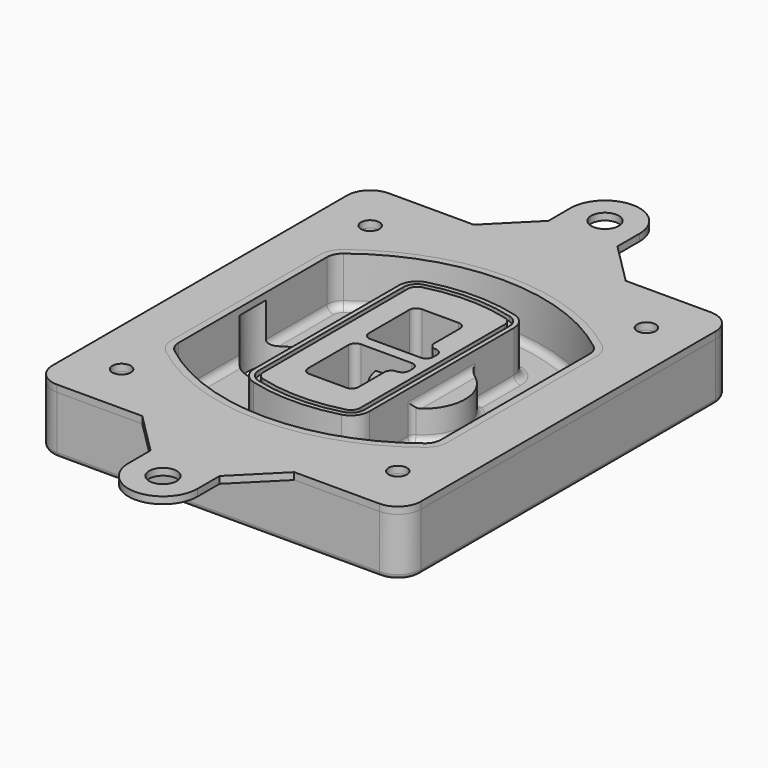
from build123d import *

# Parameters (mm, degrees)
F0_R      = 4
F1_DEPTH  = 25
F2_DEPTH  = 3
F3_DEPTH  = 18
F5_DEPTH  = 21
F6_DEPTH  = 2
F8_DEPTH  = 20
F9_DEPTH  = 16
F10_DEPTH = 25
F7_R      = 6
F7_R_2    = 4
F11_DEPTH = 6
F13_DEPTH = 9
F14_R     = 3
F15_R     = 2
F16_R     = 6
F16_R_2   = 4
F17_DEPTH = 3


# Not quite as in the source:
# - a feature names something its author has since deleted; it is built from what else it names


with BuildPart() as f1:
    # F0 (on Top) → F1 (new body)
    with BuildSketch(Plane.XY):
        with BuildLine():
            ThreePointArc((-80, -80), (-77.0710678119, -87.0710678119), (-70, -90))
            Line((-70, -90), (70, -90))
            ThreePointArc((70, -90), (77.0710678119, -87.0710678119), (80, -80))
            Line((80, -80), (80, 80))
            ThreePointArc((80, 80), (77.0710678119, 87.0710678119), (70, 90))
            Line((70, 90), (-70, 90))
            ThreePointArc((-70, 90), (-77.0710678119, 87.0710678119), (-80, 80))
            Line((-80, 80), (-80, -80))
        make_face()
        with Locations((-60, -67.5)):
            Circle(F0_R, mode=Mode.SUBTRACT)
        with Locations((60, -67.5)):
            Circle(F0_R, mode=Mode.SUBTRACT)
        with Locations((-60, 67.5)):
            Circle(F0_R, mode=Mode.SUBTRACT)
        with BuildLine():
            ThreePointArc((-64, 40.2934422872), (-62.5820384798, 46.4328484224), (-58.6153846154, 51.3286200352))
            ThreePointArc((-58.6153846154, 51.3286200352), (0, 71.5), (58.6153846154, 51.3286200352))
            ThreePointArc((58.6153846154, 51.3286200352), (62.5820384798, 46.4328484224), (64, 40.2934422872))
            Line((64, 40.2934422872), (64, -40.2934422872))
            ThreePointArc((64, -40.2934422872), (62.5820384798, -46.4328484224), (58.6153846154, -51.3286200352))
            ThreePointArc((58.6153846154, -51.3286200352), (0, -71.5), (-58.6153846154, -51.3286200352))
            ThreePointArc((-58.6153846154, -51.3286200352), (-62.5820384798, -46.4328484224), (-64, -40.2934422872))
            Line((-64, -40.2934422872), (-64, 40.2934422872))
        make_face(mode=Mode.SUBTRACT)
        with Locations((60, 67.5)):
            Circle(F0_R, mode=Mode.SUBTRACT)
        with BuildLine():
            ThreePointArc((58.6153846154, 51.3286200352), (0, 71.5), (-58.6153846154, 51.3286200352))
            ThreePointArc((-58.6153846154, 51.3286200352), (-62.5820384798, 46.4328484224), (-64, 40.2934422872))
            Line((-64, 40.2934422872), (-64, -40.2934422872))
            ThreePointArc((-64, -40.2934422872), (-62.5820384798, -46.4328484224), (-58.6153846154, -51.3286200352))
            ThreePointArc((-58.6153846154, -51.3286200352), (0, -71.5), (58.6153846154, -51.3286200352))
            ThreePointArc((58.6153846154, -51.3286200352), (62.5820384798, -46.4328484224), (64, -40.2934422872))
            Line((64, -40.2934422872), (64, 40.2934422872))
            ThreePointArc((64, 40.2934422872), (62.5820384798, 46.4328484224), (58.6153846154, 51.3286200352))
        make_face()
        with BuildLine():
            Line((-60, -40.2934422872), (-60, 40.2934422872))
            ThreePointArc((-60, 40.2934422872), (-58.9871703427, 44.6787323838), (-56.1538461538, 48.1757121072))
            ThreePointArc((-56.1538461538, 48.1757121072), (0, 67.5), (56.1538461538, 48.1757121072))
            ThreePointArc((56.1538461538, 48.1757121072), (58.9871703427, 44.6787323838), (60, 40.2934422872))
            Line((60, 40.2934422872), (60, -40.2934422872))
            ThreePointArc((60, -40.2934422872), (58.9871703427, -44.6787323838), (56.1538461538, -48.1757121072))
            ThreePointArc((56.1538461538, -48.1757121072), (0, -67.5), (-56.1538461538, -48.1757121072))
            ThreePointArc((-56.1538461538, -48.1757121072), (-58.9871703427, -44.6787323838), (-60, -40.2934422872))
        make_face(mode=Mode.SUBTRACT)
        with BuildLine():
            ThreePointArc((-56.1538461538, 48.1757121072), (-58.9871703427, 44.6787323838), (-60, 40.2934422872))
            Line((-60, 40.2934422872), (-60, -40.2934422872))
            ThreePointArc((-60, -40.2934422872), (-58.9871703427, -44.6787323838), (-56.1538461538, -48.1757121072))
            ThreePointArc((-56.1538461538, -48.1757121072), (0, -67.5), (56.1538461538, -48.1757121072))
            ThreePointArc((56.1538461538, -48.1757121072), (58.9871703427, -44.6787323838), (60, -40.2934422872))
            Line((60, -40.2934422872), (60, 40.2934422872))
            ThreePointArc((60, 40.2934422872), (58.9871703427, 44.6787323838), (56.1538461538, 48.1757121072))
            ThreePointArc((56.1538461538, 48.1757121072), (0, 67.5), (-56.1538461538, 48.1757121072))
        make_face()
        with BuildLine():
            ThreePointArc((54.3076923077, 45.8110311612), (56.2910192399, 43.3631453548), (57, 40.2934422872))
            Line((57, 40.2934422872), (57, -40.2934422872))
            ThreePointArc((57, -40.2934422872), (56.2910192399, -43.3631453548), (54.3076923077, -45.8110311612))
            ThreePointArc((54.3076923077, -45.8110311612), (0, -64.5), (-54.3076923077, -45.8110311612))
            ThreePointArc((-54.3076923077, -45.8110311612), (-56.2910192399, -43.3631453548), (-57, -40.2934422872))
            Line((-57, -40.2934422872), (-57, 40.2934422872))
            ThreePointArc((-57, 40.2934422872), (-56.2910192399, 43.3631453548), (-54.3076923077, 45.8110311612))
            ThreePointArc((-54.3076923077, 45.8110311612), (0, 64.5), (54.3076923077, 45.8110311612))
        make_face(mode=Mode.SUBTRACT)
        with BuildLine():
            Line((57, -40.2934422872), (57, 40.2934422872))
            ThreePointArc((57, 40.2934422872), (56.2910192399, 43.3631453548), (54.3076923077, 45.8110311612))
            ThreePointArc((54.3076923077, 45.8110311612), (0, 64.5), (-54.3076923077, 45.8110311612))
            ThreePointArc((-54.3076923077, 45.8110311612), (-56.2910192399, 43.3631453548), (-57, 40.2934422872))
            Line((-57, 40.2934422872), (-57, -40.2934422872))
            ThreePointArc((-57, -40.2934422872), (-56.2910192399, -43.3631453548), (-54.3076923077, -45.8110311612))
            ThreePointArc((-54.3076923077, -45.8110311612), (0, -64.5), (54.3076923077, -45.8110311612))
            ThreePointArc((54.3076923077, -45.8110311612), (56.2910192399, -43.3631453548), (57, -40.2934422872))
        make_face()
    extrude(amount=-F1_DEPTH)

    # F0 (on Top) → F2 (join)
    with BuildSketch(Plane.XY):
        with BuildLine():
            ThreePointArc((-56.1538461538, 48.1757121072), (-58.9871703427, 44.6787323838), (-60, 40.2934422872))
            Line((-60, 40.2934422872), (-60, -40.2934422872))
            ThreePointArc((-60, -40.2934422872), (-58.9871703427, -44.6787323838), (-56.1538461538, -48.1757121072))
            ThreePointArc((-56.1538461538, -48.1757121072), (0, -67.5), (56.1538461538, -48.1757121072))
            ThreePointArc((56.1538461538, -48.1757121072), (58.9871703427, -44.6787323838), (60, -40.2934422872))
            Line((60, -40.2934422872), (60, 40.2934422872))
            ThreePointArc((60, 40.2934422872), (58.9871703427, 44.6787323838), (56.1538461538, 48.1757121072))
            ThreePointArc((56.1538461538, 48.1757121072), (0, 67.5), (-56.1538461538, 48.1757121072))
        make_face()
        with BuildLine():
            ThreePointArc((54.3076923077, 45.8110311612), (56.2910192399, 43.3631453548), (57, 40.2934422872))
            Line((57, 40.2934422872), (57, -40.2934422872))
            ThreePointArc((57, -40.2934422872), (56.2910192399, -43.3631453548), (54.3076923077, -45.8110311612))
            ThreePointArc((54.3076923077, -45.8110311612), (0, -64.5), (-54.3076923077, -45.8110311612))
            ThreePointArc((-54.3076923077, -45.8110311612), (-56.2910192399, -43.3631453548), (-57, -40.2934422872))
            Line((-57, -40.2934422872), (-57, 40.2934422872))
            ThreePointArc((-57, 40.2934422872), (-56.2910192399, 43.3631453548), (-54.3076923077, 45.8110311612))
            ThreePointArc((-54.3076923077, 45.8110311612), (0, 64.5), (54.3076923077, 45.8110311612))
        make_face(mode=Mode.SUBTRACT)
    extrude(amount=F2_DEPTH)

    # F0 (on Top) → F3 (cut)
    with BuildSketch(Plane.XY):
        with BuildLine():
            Line((57, -40.2934422872), (57, 40.2934422872))
            ThreePointArc((57, 40.2934422872), (56.2910192399, 43.3631453548), (54.3076923077, 45.8110311612))
            ThreePointArc((54.3076923077, 45.8110311612), (0, 64.5), (-54.3076923077, 45.8110311612))
            ThreePointArc((-54.3076923077, 45.8110311612), (-56.2910192399, 43.3631453548), (-57, 40.2934422872))
            Line((-57, 40.2934422872), (-57, -40.2934422872))
            ThreePointArc((-57, -40.2934422872), (-56.2910192399, -43.3631453548), (-54.3076923077, -45.8110311612))
            ThreePointArc((-54.3076923077, -45.8110311612), (0, -64.5), (54.3076923077, -45.8110311612))
            ThreePointArc((54.3076923077, -45.8110311612), (56.2910192399, -43.3631453548), (57, -40.2934422872))
        make_face()
    extrude(amount=-F3_DEPTH, mode=Mode.SUBTRACT)

    # F4 (on face) → F5 (join, through all)
    with BuildSketch(Plane.XY.offset(3)):
        with BuildLine():
            ThreePointArc((-25, -39.2465276821), (-23.3511545998, -44.1109737193), (-19.0842911877, -46.9702398883))
            ThreePointArc((-19.0842911877, -46.9702398883), (0, -49.5), (19.0842911877, -46.9702398883))
            ThreePointArc((19.0842911877, -46.9702398883), (23.3511545998, -44.1109737193), (25, -39.2465276821))
            Line((25, -39.2465276821), (25, 39.2465276821))
            ThreePointArc((25, 39.2465276821), (23.3511545998, 44.1109737193), (19.0842911877, 46.9702398883))
            ThreePointArc((19.0842911877, 46.9702398883), (0, 49.5), (-19.0842911877, 46.9702398883))
            ThreePointArc((-19.0842911877, 46.9702398883), (-23.3511545998, 44.1109737193), (-25, 39.2465276821))
            Line((-25, 39.2465276821), (-25, -39.2465276821))
        make_face()
        with BuildLine():
            ThreePointArc((18.5632183908, 45.0393118368), (21.7633659499, 42.89486221), (23, 39.2465276821))
            Line((23, 39.2465276821), (23, -39.2465276821))
            ThreePointArc((23, -39.2465276821), (21.7633659499, -42.89486221), (18.5632183908, -45.0393118368))
            ThreePointArc((18.5632183908, -45.0393118368), (0, -47.5), (-18.5632183908, -45.0393118368))
            ThreePointArc((-18.5632183908, -45.0393118368), (-21.7633659499, -42.89486221), (-23, -39.2465276821))
            Line((-23, -39.2465276821), (-23, 39.2465276821))
            ThreePointArc((-23, 39.2465276821), (-21.7633659499, 42.89486221), (-18.5632183908, 45.0393118368))
            ThreePointArc((-18.5632183908, 45.0393118368), (0, 47.5), (18.5632183908, 45.0393118368))
        make_face(mode=Mode.SUBTRACT)
        with BuildLine():
            Line((23, -39.2465276821), (23, 39.2465276821))
            ThreePointArc((23, 39.2465276821), (21.7633659499, 42.89486221), (18.5632183908, 45.0393118368))
            ThreePointArc((18.5632183908, 45.0393118368), (0, 47.5), (-18.5632183908, 45.0393118368))
            ThreePointArc((-18.5632183908, 45.0393118368), (-21.7633659499, 42.89486221), (-23, 39.2465276821))
            Line((-23, 39.2465276821), (-23, -39.2465276821))
            ThreePointArc((-23, -39.2465276821), (-21.7633659499, -42.89486221), (-18.5632183908, -45.0393118368))
            ThreePointArc((-18.5632183908, -45.0393118368), (0, -47.5), (18.5632183908, -45.0393118368))
            ThreePointArc((18.5632183908, -45.0393118368), (21.7633659499, -42.89486221), (23, -39.2465276821))
        make_face()
        with BuildLine():
            ThreePointArc((18.0421455939, 43.1083837852), (20.1755772999, 41.6787507007), (21, 39.2465276821))
            Line((21, 39.2465276821), (21, -39.2465276821))
            ThreePointArc((21, -39.2465276821), (20.1755772999, -41.6787507007), (18.0421455939, -43.1083837852))
            ThreePointArc((18.0421455939, -43.1083837852), (0, -45.5), (-18.0421455939, -43.1083837852))
            ThreePointArc((-18.0421455939, -43.1083837852), (-20.1755772999, -41.6787507007), (-21, -39.2465276821))
            Line((-21, -39.2465276821), (-21, 39.2465276821))
            ThreePointArc((-21, 39.2465276821), (-20.1755772999, 41.6787507007), (-18.0421455939, 43.1083837852))
            ThreePointArc((-18.0421455939, 43.1083837852), (0, 45.5), (18.0421455939, 43.1083837852))
        make_face(mode=Mode.SUBTRACT)
        with BuildLine():
            Line((21, -39.2465276821), (21, 39.2465276821))
            ThreePointArc((21, 39.2465276821), (20.1755772999, 41.6787507007), (18.0421455939, 43.1083837852))
            ThreePointArc((18.0421455939, 43.1083837852), (0, 45.5), (-18.0421455939, 43.1083837852))
            ThreePointArc((-18.0421455939, 43.1083837852), (-20.1755772999, 41.6787507007), (-21, 39.2465276821))
            Line((-21, 39.2465276821), (-21, -39.2465276821))
            ThreePointArc((-21, -39.2465276821), (-20.1755772999, -41.6787507007), (-18.0421455939, -43.1083837852))
            ThreePointArc((-18.0421455939, -43.1083837852), (0, -45.5), (18.0421455939, -43.1083837852))
            ThreePointArc((18.0421455939, -43.1083837852), (20.1755772999, -41.6787507007), (21, -39.2465276821))
        make_face()
        with BuildLine():
            Line((-8, -2.5), (14, -2.5))
            ThreePointArc((14, -2.5), (16.1213203436, -3.3786796564), (17, -5.5))
            Line((17, -5.5), (17, -7.5))
            ThreePointArc((17, -7.5), (16.1213203436, -9.6213203436), (14, -10.5))
            ThreePointArc((14, -10.5), (11.8786796564, -11.3786796564), (11, -13.5))
            Line((11, -13.5), (11, -27.5))
            ThreePointArc((11, -27.5), (10.1213203436, -29.6213203436), (8, -30.5))
            Line((8, -30.5), (-8, -30.5))
            ThreePointArc((-8, -30.5), (-10.1213203436, -29.6213203436), (-11, -27.5))
            Line((-11, -27.5), (-11, -5.5))
            ThreePointArc((-11, -5.5), (-10.1213203436, -3.3786796564), (-8, -2.5))
        make_face(mode=Mode.SUBTRACT)
        with BuildLine():
            ThreePointArc((-8, 2.5), (-10.1213203436, 3.3786796564), (-11, 5.5))
            Line((-11, 5.5), (-11, 27.5))
            ThreePointArc((-11, 27.5), (-10.1213203436, 29.6213203436), (-8, 30.5))
            Line((-8, 30.5), (8, 30.5))
            ThreePointArc((8, 30.5), (10.1213203436, 29.6213203436), (11, 27.5))
            Line((11, 27.5), (11, 13.5))
            ThreePointArc((11, 13.5), (11.8786796564, 11.3786796564), (14, 10.5))
            ThreePointArc((14, 10.5), (16.1213203436, 9.6213203436), (17, 7.5))
            Line((17, 7.5), (17, 5.5))
            ThreePointArc((17, 5.5), (16.1213203436, 3.3786796564), (14, 2.5))
            Line((14, 2.5), (-8, 2.5))
        make_face(mode=Mode.SUBTRACT)
    extrude(amount=-F5_DEPTH)

    # F4 (on face) → F6 (cut)
    with BuildSketch(Plane.XY.offset(3)):
        with BuildLine():
            Line((23, -39.2465276821), (23, 39.2465276821))
            ThreePointArc((23, 39.2465276821), (21.7633659499, 42.89486221), (18.5632183908, 45.0393118368))
            ThreePointArc((18.5632183908, 45.0393118368), (0, 47.5), (-18.5632183908, 45.0393118368))
            ThreePointArc((-18.5632183908, 45.0393118368), (-21.7633659499, 42.89486221), (-23, 39.2465276821))
            Line((-23, 39.2465276821), (-23, -39.2465276821))
            ThreePointArc((-23, -39.2465276821), (-21.7633659499, -42.89486221), (-18.5632183908, -45.0393118368))
            ThreePointArc((-18.5632183908, -45.0393118368), (0, -47.5), (18.5632183908, -45.0393118368))
            ThreePointArc((18.5632183908, -45.0393118368), (21.7633659499, -42.89486221), (23, -39.2465276821))
        make_face()
        with BuildLine():
            ThreePointArc((18.0421455939, 43.1083837852), (20.1755772999, 41.6787507007), (21, 39.2465276821))
            Line((21, 39.2465276821), (21, -39.2465276821))
            ThreePointArc((21, -39.2465276821), (20.1755772999, -41.6787507007), (18.0421455939, -43.1083837852))
            ThreePointArc((18.0421455939, -43.1083837852), (0, -45.5), (-18.0421455939, -43.1083837852))
            ThreePointArc((-18.0421455939, -43.1083837852), (-20.1755772999, -41.6787507007), (-21, -39.2465276821))
            Line((-21, -39.2465276821), (-21, 39.2465276821))
            ThreePointArc((-21, 39.2465276821), (-20.1755772999, 41.6787507007), (-18.0421455939, 43.1083837852))
            ThreePointArc((-18.0421455939, 43.1083837852), (0, 45.5), (18.0421455939, 43.1083837852))
        make_face(mode=Mode.SUBTRACT)
    extrude(amount=-F6_DEPTH, mode=Mode.SUBTRACT)

    # F7 (on face) → F8 (join)
    with BuildSketch(Plane(origin=(0, 0, -25), x_dir=(1, 0, 0), z_dir=(0, 0, -1))):
        with BuildLine():
            ThreePointArc((3.28842436, 0), (16.7567035675, 13.4682792075), (30.224982775, 0))
            Line((30.224982775, 0), (35.224982775, 0))
            ThreePointArc((35.224982775, 0), (16.7567035675, 18.4682792075), (-1.71157564, 0))
            Line((-1.71157564, 0), (3.28842436, 0))
        make_face()
        with BuildLine():
            Line((3.28842436, 0), (30.224982775, 0))
            ThreePointArc((30.224982775, 0), (16.7567035675, 13.4682792075), (3.28842436, 0))
        make_face()
        with BuildLine():
            ThreePointArc((3.28842436, 0), (16.7567035675, -13.4682792075), (30.224982775, 0))
            Line((30.224982775, 0), (3.28842436, 0))
        make_face()
        with BuildLine():
            Line((35.224982775, 0), (30.224982775, 0))
            ThreePointArc((30.224982775, 0), (16.7567035675, -13.4682792075), (3.28842436, 0))
            Line((3.28842436, 0), (-1.71157564, 0))
            ThreePointArc((-1.71157564, 0), (16.7567035675, -18.4682792075), (35.224982775, 0))
        make_face()
    extrude(amount=-F8_DEPTH)

    # F7 (on face) → F9 (cut)
    with BuildSketch(Plane(origin=(0, 0, -25), x_dir=(1, 0, 0), z_dir=(0, 0, -1))):
        with BuildLine():
            Line((3.28842436, 0), (30.224982775, 0))
            ThreePointArc((30.224982775, 0), (16.7567035675, 13.4682792075), (3.28842436, 0))
        make_face()
        with BuildLine():
            ThreePointArc((3.28842436, 0), (16.7567035675, -13.4682792075), (30.224982775, 0))
            Line((30.224982775, 0), (3.28842436, 0))
        make_face()
    extrude(amount=-F9_DEPTH, mode=Mode.SUBTRACT)

    # F7 (on face) → F10 (cut)
    with BuildSketch(Plane(origin=(0, 0, -25), x_dir=(1, 0, 0), z_dir=(0, 0, -1))):
        with BuildLine():
            Line((-59.0318229325, 0), (-32.0952645175, 0))
            ThreePointArc((-32.0952645175, 0), (-45.563543725, 13.4682792075), (-59.0318229325, 0))
        make_face()
        with BuildLine():
            ThreePointArc((-59.0318229325, 0), (-45.563543725, -13.4682792075), (-32.0952645175, 0))
            Line((-32.0952645175, 0), (-59.0318229325, 0))
        make_face()
    extrude(amount=-F10_DEPTH, mode=Mode.SUBTRACT)

    # F7 (on face) → F11 (cut)
    with BuildSketch(Plane(origin=(0, 0, -25), x_dir=(1, 0, 0), z_dir=(0, 0, -1))):
        with Locations((60, -67.5)):
            Circle(F7_R)
        with Locations((60, -67.5)):
            Circle(F7_R_2, mode=Mode.SUBTRACT)
        with Locations((-60, -67.5)):
            Circle(F7_R)
        with Locations((-60, -67.5)):
            Circle(F7_R_2, mode=Mode.SUBTRACT)
        with Locations((-60, 67.5)):
            Circle(F7_R)
        with Locations((-60, 67.5)):
            Circle(F7_R_2, mode=Mode.SUBTRACT)
        with Locations((60, 67.5)):
            Circle(F7_R)
        with Locations((60, 67.5)):
            Circle(F7_R_2, mode=Mode.SUBTRACT)
    extrude(amount=-F11_DEPTH, mode=Mode.SUBTRACT)

    # F12 (on face) → F13 (cut, through all)
    with BuildSketch(Plane(origin=(0, 0, -9), x_dir=(1, 0, 0), z_dir=(0, 0, -1))):
        with BuildLine():
            Line((11, 13.5), (11, 17.5481537753))
            ThreePointArc((11, 17.5481537753), (2.5696536419, 11.8239143813), (-1.5415842455, 2.5))
            Line((-1.5415842455, 2.5), (3.5224848595, 2.5))
            ThreePointArc((3.5224848595, 2.5), (6.1857188154, 8.3455872281), (11.2536447004, 12.2927168648))
            ThreePointArc((11.2536447004, 12.2927168648), (11.0640958889, 12.8831798879), (11, 13.5))
        make_face()
        with BuildLine():
            ThreePointArc((11.2536447004, -12.2927168648), (6.1857188154, -8.3455872281), (3.5224848595, -2.5))
            Line((3.5224848595, -2.5), (-1.5415842455, -2.5))
            ThreePointArc((-1.5415842455, -2.5), (2.5696536419, -11.8239143813), (11, -17.5481537753))
            Line((11, -17.5481537753), (11, -13.5))
            ThreePointArc((11, -13.5), (11.0640958889, -12.8831798879), (11.2536447004, -12.2927168648))
        make_face()
        with BuildLine():
            ThreePointArc((11.2536447004, 12.2927168648), (6.1857188154, 8.3455872281), (3.5224848595, 2.5))
            Line((3.5224848595, 2.5), (14, 2.5))
            ThreePointArc((14, 2.5), (16.1213203436, 3.3786796564), (17, 5.5))
            Line((17, 5.5), (17, 7.5))
            ThreePointArc((17, 7.5), (16.1213203436, 9.6213203436), (14, 10.5))
            ThreePointArc((14, 10.5), (12.3601599782, 10.9878446101), (11.2536447004, 12.2927168648))
        make_face()
        with BuildLine():
            Line((14, -2.5), (3.5224848595, -2.5))
            ThreePointArc((3.5224848595, -2.5), (6.1857188154, -8.3455872281), (11.2536447004, -12.2927168648))
            ThreePointArc((11.2536447004, -12.2927168648), (12.3601599782, -10.9878446101), (14, -10.5))
            ThreePointArc((14, -10.5), (16.1213203436, -9.6213203436), (17, -7.5))
            Line((17, -7.5), (17, -5.5))
            ThreePointArc((17, -5.5), (16.1213203436, -3.3786796564), (14, -2.5))
        make_face()
    extrude(amount=F13_DEPTH, mode=Mode.SUBTRACT)

    # F14
    f14_edges = [f1.edges().sort_by_distance(p)[0] for p in [
        (-57, -23.703476, -18),
        (-57, 23.703476, -18),
        (25, 0, -5),
        (25, 16.526506, -11.5),
        (25, -16.526506, -11.5),
        (25, -27.886517, -18),
        (35.224983, 0, -18),
    ]]
    fillet(f14_edges, radius=F14_R)

    # F15
    f15_edges = [f1.edges().sort_by_distance(p)[0] for p in [
        (0, -90, -25),
    ]]
    fillet(f15_edges, radius=F15_R)


with BuildPart() as f17:
    # F16 (on face) → F17 (new body, through all)
    with BuildSketch(Plane.XY):
        with BuildLine():
            Line((-15, 108), (-33, 90))
            Line((-33, 90), (33, 90))
            Line((33, 90), (15, 108))
            Line((15, 108), (15, 120))
            ThreePointArc((15, 120), (0, 135), (-15, 120))
            Line((-15, 120), (-15, 108))
        make_face()
        with Locations((0, 120)):
            Circle(F16_R, mode=Mode.SUBTRACT)
        with BuildLine():
            Line((33, 90), (-33, 90))
            Line((-33, 90), (-70, 90))
            ThreePointArc((-70, 90), (-77.0710678119, 87.0710678119), (-80, 80))
            Line((-80, 80), (-80, -80))
            ThreePointArc((-80, -80), (-77.0710678119, -87.0710678119), (-70, -90))
            Line((-70, -90), (-33, -90))
            Line((-33, -90), (33, -90))
            Line((33, -90), (70, -90))
            ThreePointArc((70, -90), (77.0710678119, -87.0710678119), (80, -80))
            Line((80, -80), (80, 80))
            ThreePointArc((80, 80), (77.0710678119, 87.0710678119), (70, 90))
            Line((70, 90), (33, 90))
        make_face()
        with Locations((-60, -67.5)):
            Circle(F16_R_2, mode=Mode.SUBTRACT)
        with BuildLine():
            ThreePointArc((-60, 40.2934422872), (-58.9871703427, 44.6787323838), (-56.1538461538, 48.1757121072))
            ThreePointArc((-56.1538461538, 48.1757121072), (0, 67.5), (56.1538461538, 48.1757121072))
            ThreePointArc((56.1538461538, 48.1757121072), (58.9871703427, 44.6787323838), (60, 40.2934422872))
            Line((60, 40.2934422872), (60, -40.2934422872))
            ThreePointArc((60, -40.2934422872), (58.9871703427, -44.6787323838), (56.1538461538, -48.1757121072))
            ThreePointArc((56.1538461538, -48.1757121072), (0, -67.5), (-56.1538461538, -48.1757121072))
            ThreePointArc((-56.1538461538, -48.1757121072), (-58.9871703427, -44.6787323838), (-60, -40.2934422872))
            Line((-60, -40.2934422872), (-60, 40.2934422872))
        make_face(mode=Mode.SUBTRACT)
        with Locations((60, -67.5)):
            Circle(F16_R_2, mode=Mode.SUBTRACT)
        with Locations((-60, 67.5)):
            Circle(F16_R_2, mode=Mode.SUBTRACT)
        with Locations((60, 67.5)):
            Circle(F16_R_2, mode=Mode.SUBTRACT)
        with BuildLine():
            Line((33, -90), (-33, -90))
            Line((-33, -90), (-15, -108))
            Line((-15, -108), (-15, -120))
            ThreePointArc((-15, -120), (0, -135), (15, -120))
            Line((15, -120), (15, -108))
            Line((15, -108), (33, -90))
        make_face()
        with Locations((0, -120)):
            Circle(F16_R, mode=Mode.SUBTRACT)
    extrude(amount=F17_DEPTH)


solid = Compound([f1.part, f17.part])
